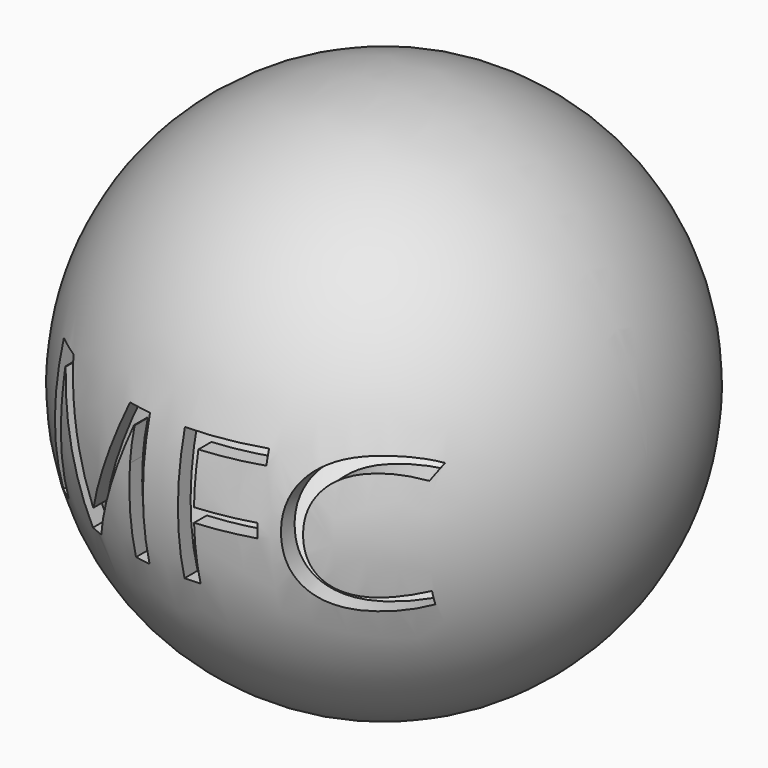
from build123d import *

# Parameters (mm, degrees)
F2_TEXT_SIZE = 35.2822606348
F3_DEPTH     = 50.001


# Not quite as in the source:
# - Text() gives the source's letters only with a copy of the font that has no kerning and outlines rounded to 1/6400 em; it was checked with that copy


with BuildPart() as f1:
    # F0 (on Front) → F1 (revolve)
    with BuildSketch(Plane.XZ):
        with BuildLine():
            Line((47, 0), (50, 0))
            ThreePointArc((50, 0), (0, 50), (-50, 0))
            Line((-50, 0), (-47, 0))
            ThreePointArc((-47, 0), (0, 47), (47, 0))
        make_face()
    revolve(axis=Axis((-25, 0, 0), (-1, 0, 0)))

    # F2 (on Front) → F3 (cut, through all)
    with BuildSketch(Plane.XZ):
        with Locations((-34.3690724112, -12.4027524143)):
            Text('MFC', F2_TEXT_SIZE, font='Open Sans', text_align=(TextAlign.LEFT, TextAlign.BOTTOM))
    extrude(amount=F3_DEPTH, mode=Mode.SUBTRACT)


solid = f1.part
